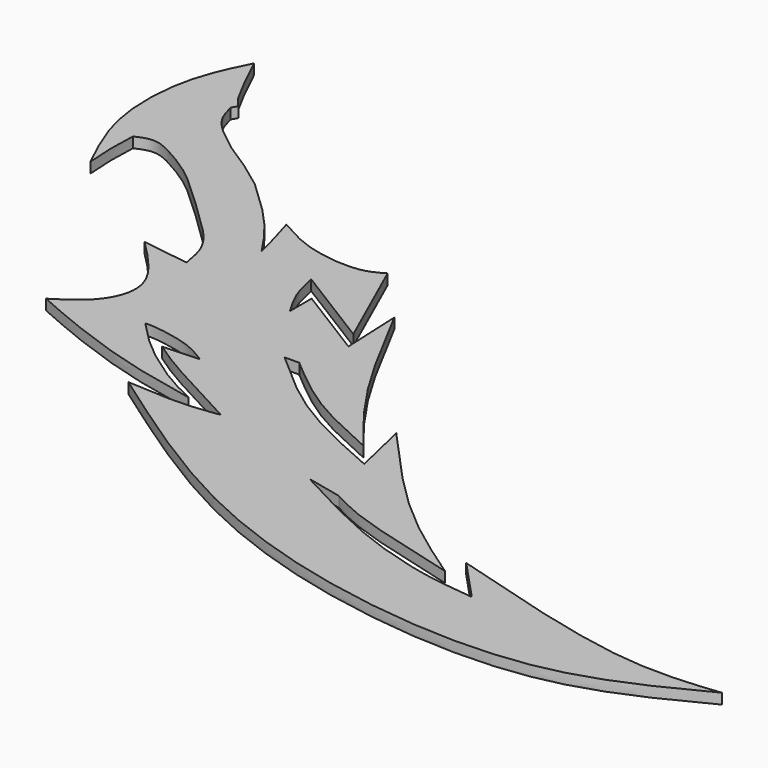
from build123d import *

# Parameters (mm, degrees)
F1_DEPTH = 1


# Not quite as in the source:
# - a feature names something its author has since deleted; it is built from what else it names


with BuildPart() as f1:
    # F0 (on Top) → F1 (new body)
    with BuildSketch(Plane.XY):
        with BuildLine():
            add(Edge.make_bspline(
                [(-16.6099965572, 10.2172633633), (-15.4212118205, 9.5285409053), (-12.9551826674, 8.0998468723), (-7.766656534, 7.5933629956), (-6.3511176621, 8.4439850217), (-5.7889274321, 8.7818149477)],
                knots=[0, 0, 0, 0, 0.3594226743, 0.7455906573, 1, 1, 1, 1], degree=3))
            add(Edge.make_bspline(
                [(-16.6099965572, 10.2172633633), (-16.3713958805, 9.4307097449), (-15.904194945, 7.8905691575), (-15.5435341339, 6.4249386215), (-15.3670636937, 5.7078092359)],
                knots=[0, 0, 0, 0, 0.5107024806, 1, 1, 1, 1], degree=3))
            add(Edge.make_bspline(
                [(-22.5439389952, 13.8567826848), (-20.9328268461, 12.3755889493), (-17.8750260099, 9.497072632), (-16.1981091624, 6.9589873468), (-15.3670636937, 5.7078092359)],
                knots=[0.1092468408, 0.1092468408, 0.1092468408, 0.1092468408, 0.5599397099, 1, 1, 1, 1], degree=3))
            add(Edge.make_bspline(
                [(-24.9835465397, 15.6512659715), (-24.5105414607, 15.2932659882), (-23.6115055046, 14.644329683), (-22.8821580713, 14.1081462449), (-22.5439389952, 13.8567826848)],
                knots=[0, 0, 0, 0, 0.5340013105, 1, 1, 1, 1], degree=3))
            add(Edge.make_bspline(
                [(-31.6534787416, 22.3535578698), (-31.4894436188, 21.7239753561), (-31.1336922454, 20.3585675093), (-29.1441485457, 18.4393483759), (-26.688509429, 16.66011353), (-24.9835465397, 15.6512659715)],
                knots=[0, 0, 0, 0, 0.1581489893, 0.342985814, 0.5895394489, 0.5895394489, 0.5895394489, 0.5895394489], degree=3))
            Line((-31.6534787416, 22.3535578698), (-31.3492268324, 22.8967126459))
            add(Edge.make_bspline(
                [(-34.7586423159, 29.0321223438), (-34.3418990536, 28.1776650529), (-33.5153831208, 26.4830424187), (-32.2770591236, 23.9047003589), (-31.6167279276, 23.1873231579), (-31.3492268324, 22.8967126459)],
                knots=[0, 0, 0, 0, 0.3769541602, 0.747603255, 1, 1, 1, 1], degree=3))
            add(Edge.make_bspline(
                [(-34.7586423159, 29.0321223438), (-35.5677944518, 27.4079633385), (-37.3288786405, 23.8782557478), (-37.627728367, 15.760880925), (-35.454224769, 11.2387606607), (-34.3599178116, 9.002301842)],
                knots=[0, 0, 0, 0, 0.3007790413, 0.6538294353, 1, 1, 1, 1], degree=3))
            add(Edge.make_bspline(
                [(-34.3599178116, 9.002301842), (-34.4460411955, 10.0396901503), (-34.5463298451, 11.768741471), (-34.4792390008, 13.4920788706), (-34.4357995181, 14.1820461029)],
                knots=[0, 0, 0, 0, 0.5004169403, 0.8340605609, 0.8340605609, 0.8340605609, 0.8340605609], degree=3))
            add(Edge.make_bspline(
                [(-18.5956805944, 0.7639901596), (-18.754914474, 1.762296212), (-19.1182465354, 4.0401820297), (-22.8890828074, 7.5134991963), (-26.9671489576, 11.505197563), (-29.4215545254, 13.182958406), (-32.0236221513, 14.6651885876), (-33.3319524476, 14.6676349212), (-34.0719301846, 14.3425994686), (-34.4357995181, 14.1820461029)],
                knots=[0, 0, 0, 0, 0.1460617246, 0.3332764838, 0.5324015784, 0.6782952182, 0.8179917645, 0.9100820113, 0.9991741954, 0.9991741954, 0.9991741954, 0.9991741954], degree=3))
            add(Edge.make_bspline(
                [(-23.1238305569, 1.4212612296), (-22.2308115866, 1.302547656), (-20.5628255796, 1.0808137554), (-19.2197091749, 0.8644946878), (-18.5956805944, 0.7639901596)],
                knots=[0, 0, 0, 0, 0.5353875671, 1, 1, 1, 1], degree=3))
            add(Edge.make_bspline(
                [(-23.1238305569, -10.3354090825), (-21.9181343668, -9.5672404628), (-19.5647077627, -8.0678341604), (-18.0730916869, -3.6305347437), (-21.2811829424, -0.4217720451), (-23.1238305569, 1.4212612296)],
                knots=[0, 0, 0, 0, 0.3089727792, 0.603091197, 1, 1, 1, 1], degree=3))
            add(Edge.make_bspline(
                [(-4.8519154079, -16.1593034863), (-7.4154305721, -15.6333116353), (-12.4370011009, -14.6029665784), (-19.2999839188, -12.0288214544), (-21.9779293524, -10.8428779902), (-23.1238305569, -10.3354090825)],
                knots=[0, 0, 0, 0, 0.3736855161, 0.7319980787, 1, 1, 1, 1], degree=3))
            add(Edge.make_bspline(
                [(-14.8473009467, -8.831509389), (-14.0171136981, -9.7171202904), (-12.2176917006, -11.6366724638), (-7.9071133303, -14.7016545165), (-5.7918028227, -15.7108788812), (-4.8519154079, -16.1593034863)],
                knots=[0, 0, 0, 0, 0.322473213, 0.6989572463, 1, 1, 1, 1], degree=3))
            add(Edge.make_bspline(
                [(-8.0227525905, -10.816199705), (-8.7445347825, -10.3543101709), (-10.2936553467, -9.3629826161), (-14.0342744282, -8.7559960985), (-14.6547502449, -8.8136254249), (-14.8473009467, -8.831509389)],
                knots=[0, 0, 0, 0, 0.3756557433, 0.806248815, 1, 1, 1, 1], degree=3))
            Line((-8.0227525905, -10.816199705), (-11.5278782323, -10.9786894172))
            add(Edge.make_bspline(
                [(-1.2948540742, -16.8027080712), (-4.3131749279, -15.2063237418), (-9.020596995, -12.7165640866), (-10.8657693402, -11.4376176997), (-11.5278782323, -10.9786894172)],
                knots=[4.22789e-05, 4.22789e-05, 4.22789e-05, 4.22789e-05, 0.6411820822, 1, 1, 1, 1], degree=3))
            add(Edge.make_bspline(
                [(-9.9178981036, -17.0243084431), (-8.0369774486, -17.152822121), (-4.8078227744, -17.3734537264), (-1.2910580124, -16.912451153), (-1.2927963607, -16.8091016917), (-1.2948540742, -16.8027080712)],
                knots=[0, 0, 0, 0, 0.5593319314, 0.960258114, 0.9872401448, 0.9872401448, 0.9872401448, 0.9872401448], degree=3))
            add(Edge.make_bspline(
                [(56.0104735196, -28.554501012), (51.9388012895, -30.6732939687), (43.1626287248, -35.2401872663), (23.7757696907, -34.1342565116), (6.1000439104, -28.3431760834), (-4.5392052922, -20.825090838), (-9.9178981036, -17.0243084431)],
                knots=[0, 0, 0, 0, 0.2229662615, 0.4805864215, 0.7374094706, 1, 1, 1, 1], degree=3))
            add(Edge.make_bspline(
                [(28.0218664557, -24.0996014327), (34.8843220952, -26.1370758676), (46.4307325782, -29.5652242463), (53.2458361821, -28.8461877297), (56.0104735196, -28.554501012)],
                knots=[0, 0, 0, 0, 0.5943367118, 1, 1, 1, 1], degree=3))
            Line((28.0218664557, -24.0996014327), (31.7761152983, -28.129896149))
            add(Edge.make_bspline(
                [(10.4167964309, -20.7992941141), (13.3020900166, -22.350921559), (18.7887841643, -25.301506991), (26.4258501352, -27.584558387), (30.1169773998, -27.9607848021), (31.7761152983, -28.129896149)],
                knots=[0, 0, 0, 0, 0.3791070825, 0.7209126382, 1, 1, 1, 1], degree=3))
            Line((10.4167964309, -20.7992941141), (13.8279302046, -21.5669311583))
            add(Edge.make_bspline(
                [(27.6213772595, -26.1221751571), (23.6067244924, -25.076781429), (17.2832552929, -23.4301844692), (14.7521015867, -22.0652823535), (13.8279302046, -21.5669311583)],
                knots=[0, 0, 0, 0, 0.6348813666, 1, 1, 1, 1], degree=3))
            add(Edge.make_bspline(
                [(10.8465477824, -10.9871085733), (13.7292478088, -14.2236435187), (19.1884297009, -20.3529087233), (24.9175139429, -24.2723702383), (27.6213772595, -26.1221751571)],
                knots=[0, 0, 0, 0, 0.5280461584, 1, 1, 1, 1], degree=3))
            Line((10.8465477824, -10.9871085733), (12.0913498104, -16.3664314896))
            add(Edge.make_bspline(
                [(-3.3141928725, -6.6230124794), (-1.2243299559, -8.513743245), (3.1043671989, -12.4299813966), (9.0277383612, -15.0245179581), (12.0913498104, -16.3664314896)],
                knots=[0, 0, 0, 0, 0.4827925914, 1, 1, 1, 1], degree=3))
            Line((-3.3141928725, -6.6230124794), (-1.909304643, -6.6230124794))
            add(Edge.make_bspline(
                [(10.2238217369, -14.115748927), (7.8172960071, -13.0456945157), (3.181551384, -10.9844246435), (-0.2561811543, -8.0392679882), (-1.909304643, -6.6230124794)],
                knots=[0, 0, 0, 0, 0.5191238788, 1, 1, 1, 1], degree=3))
            add(Edge.make_bspline(
                [(-0.9440209251, 3.5210286733), (1.0464920899, -0.3056682218), (4.6957007503, -7.3211538505), (8.4963093931, -11.9924692639), (10.2238217369, -14.115748927)],
                knots=[0, 0, 0, 0, 0.5454642911, 1, 1, 1, 1], degree=3))
            Line((-0.9440209251, 3.5210286733), (-0.6881441002, -2.2778437083))
            Line((-0.6881441002, -2.2778437083), (-7.6660518534, 2.0532717463))
            Line((-7.6660518534, 2.0532717463), (-7.6660518534, -0.5485964357))
            add(Edge.make_bspline(
                [(-9.6535952762, 4.4754715636), (-9.4700688508, 3.6180804257), (-9.0971451505, 1.8758709595), (-8.1480633424, 0.2679968231), (-7.6660518534, -0.5485964357)],
                knots=[0, 0, 0, 0, 0.4921286186, 1, 1, 1, 1], degree=3))
            Line((-9.6535952762, 4.4754715636), (-1.648212783, -0.4933868768))
            Line((-1.648212783, -0.4933868768), (-5.7889274321, 8.7818149477))
        make_face()
    extrude(amount=F1_DEPTH)


solid = f1.part
